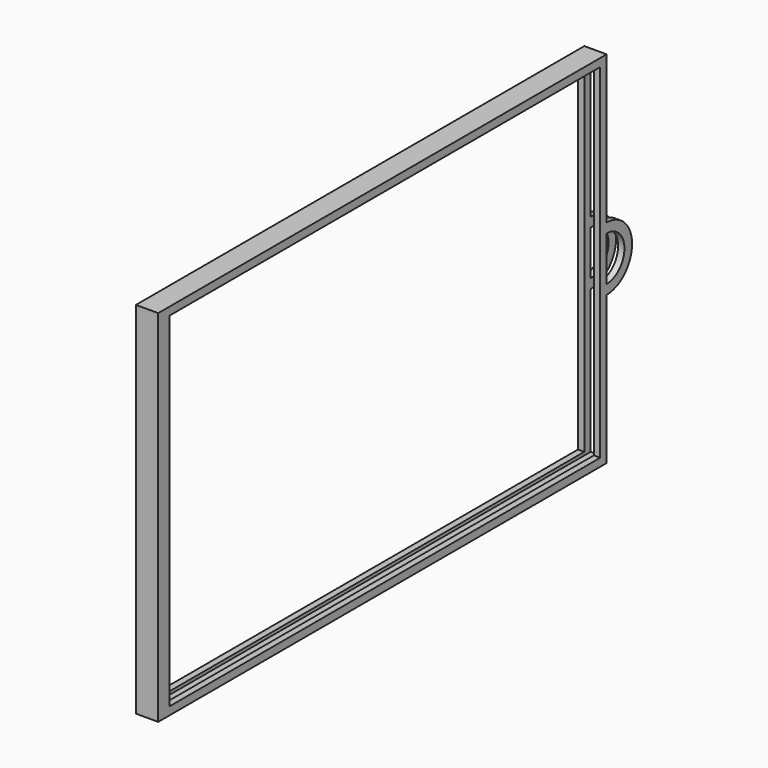
from build123d import *

# Parameters (mm, degrees)
F1_DEPTH      = 1.75
F2_W          = 1.5
F2_H          = 55
F3_DEPTH      = 43.25
F3_DEPTH_BACK = 58.6


with BuildPart() as f1:
    # F0 (on Right) → F1 (new body, symmetric)
    with BuildSketch(Plane.YZ):
        Polygon((-42.75, -27), (-42.75, 27), (-41.75, 27), (-41.75, 28.25), (-44, 28.25), (-44, -28.25), (-41.75, -28.25), (-41.75, -27), align=None)
        Polygon((-41.75, 27), (-42.75, 27), (-42.75, -27), (-41.75, -27), (-41.75, -26), (-41.75, 26), align=None)
        Polygon((-41.75, 28.25), (-41.75, 27), (42.75, 27), (42.75, -27), (-41.75, -27), (-41.75, -28.25), (44, -28.25), (44, -5), (44, -3.5), (44, 3.5), (44, 5), (44, 28.25), align=None)
        with BuildLine():
            ThreePointArc((44, -5), (49, 0), (44, 5))
            Line((44, 5), (44, 3.5))
            ThreePointArc((44, 3.5), (47.5, 0), (44, -3.5))
            Line((44, -3.5), (44, -5))
        make_face()
    extrude(amount=F1_DEPTH, both=True)

    # F2 (on Front) → F3 (cut, two sides)
    with BuildSketch(Plane.XZ) as f3_sk:
        Rectangle(F2_W, F2_H)
    extrude(amount=F3_DEPTH, mode=Mode.SUBTRACT)
    extrude(f3_sk.sketch, amount=-F3_DEPTH_BACK, mode=Mode.SUBTRACT)


solid = f1.part
